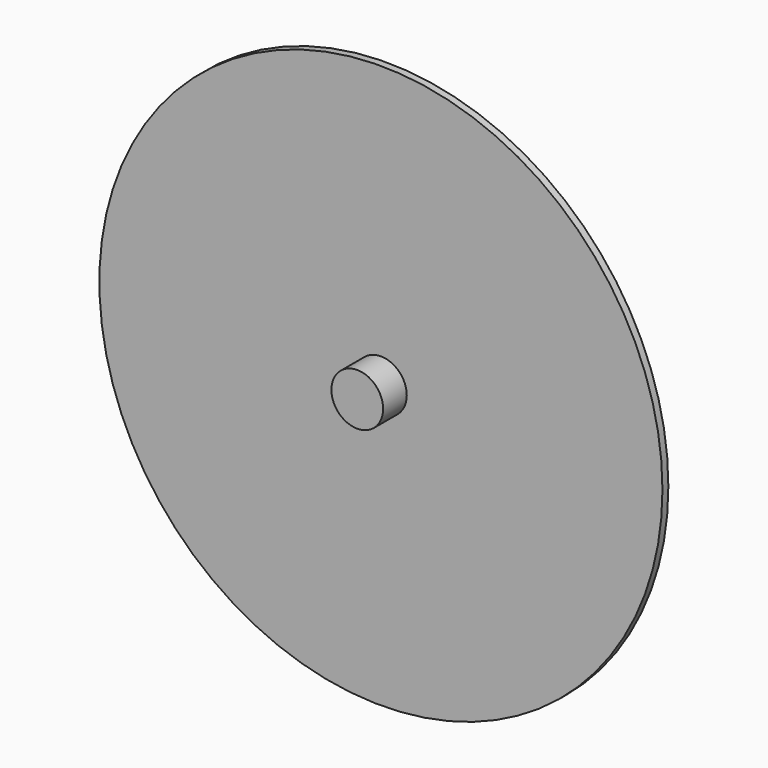
from build123d import *

# Parameters (mm, degrees)
F0_R     = 38.1
F1_DEPTH = 1
F2_R     = 3.5
F3_DEPTH = 4


# Not quite as in the source:
# - a feature of the source that left no trace in its solid (it failed there, or was rolled back) is left out
# - the program builds the solid bodies; features that only make, move or delete a surface that nothing else refers to are left out


with BuildPart() as f1:
    # F0 (on Front) → F1 (new body)
    with BuildSketch(Plane.XZ):
        with Locations((-7.189839147, 7.005484309)):
            Circle(F0_R)
    extrude(amount=F1_DEPTH)

    # F2 (on face) → F3 (join)
    with BuildSketch(Plane.XZ.offset(1)):
        with Locations((-7.189839147, 7.005484309)):
            Circle(F2_R)
    extrude(amount=F3_DEPTH)


solid = f1.part
